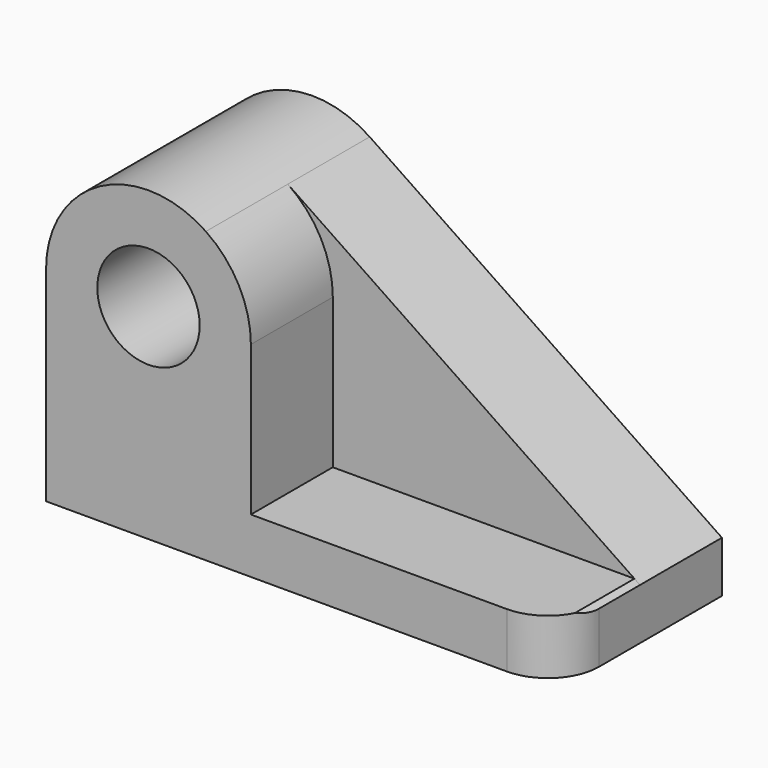
from build123d import *

# Parameters (mm, degrees)
F0_R     = 12.7
F1_DEPTH = 25.4
F2_R     = 12.7
F3_DEPTH = 25.4
F4_R     = 12.7


# Not quite as in the source:
# - ends of sketch curves that miss each other by under 0.0002 mm in the source are joined


with BuildPart() as f1:
    # F0 (on Front) → F1 (new body)
    with BuildSketch(Plane.XZ):
        with BuildLine():
            Line((40.9585287035, -61.2564672112), (-46.4072367427, -2.1416516533))
            ThreePointArc((-46.4072367427, -2.1416516533), (-72.5399719473, -0.7377161417), (-86.0414712965, -23.1564672112))
            ThreePointArc((-86.0414712965, -23.1564672112), (-86.041478422, -23.1674516111), (-86.0414807971, -23.1784360131))
            Line((-86.0414807971, -23.1784360131), (-86.0414712965, -73.9564672112))
            Line((-86.0414712965, -73.9564672112), (40.9585287035, -73.9564672112))
            Line((40.9585287035, -73.9564672112), (40.9585287035, -61.2564672112))
        make_face()
        with Locations((-60.6414807971, -23.1784360131)):
            Circle(F0_R, mode=Mode.SUBTRACT)
    extrude(amount=F1_DEPTH)

    # F2 (on face) → F3 (join)
    with BuildSketch(Plane.XZ.offset(25.4)):
        with BuildLine():
            Line((-35.2414807971, -60.323882848), (-35.2414807971, -23.1784360131))
            ThreePointArc((-35.2414807971, -23.1784360131), (-38.2059086071, -11.2702413343), (-46.4072367427, -2.1416516533))
            ThreePointArc((-46.4072367427, -2.1416516533), (-72.5399719473, -0.7377161417), (-86.0414712965, -23.1564672112))
            ThreePointArc((-86.0414712965, -23.1564672112), (-86.041478422, -23.1674516111), (-86.0414807971, -23.1784360131))
            Line((-86.0414807971, -23.1784360131), (-86.0414712965, -60.323882848))
            Line((-86.0414712965, -60.323882848), (-86.0414712965, -73.9564672112))
            Line((-86.0414712965, -73.9564672112), (40.9585287035, -73.9564672112))
            Line((40.9585287035, -73.9564672112), (40.9585287035, -61.2564672112))
            Line((40.9585287035, -61.2564672112), (39.5802625959, -60.323882848))
            Line((39.5802625959, -60.323882848), (-35.2414807971, -60.323882848))
        make_face()
        with Locations((-60.6414807971, -23.1784360131)):
            Circle(F2_R, mode=Mode.SUBTRACT)
    extrude(amount=F3_DEPTH)

    # F4
    f4_edges = [f1.edges().sort_by_distance(p)[0] for p in [
        (40.958529, -50.8, -67.606467),
    ]]
    fillet(f4_edges, radius=F4_R)


solid = f1.part
